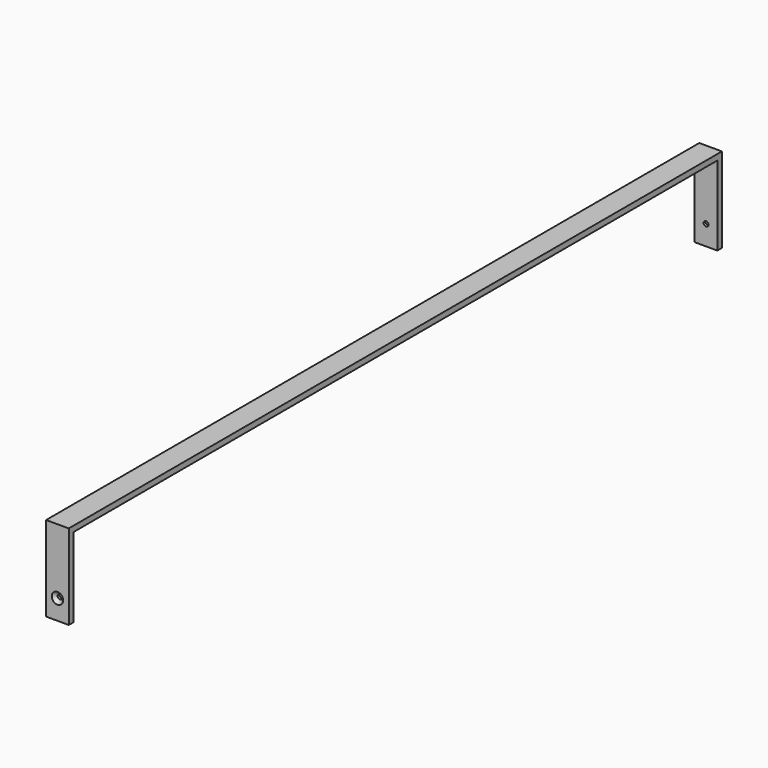
from build123d import *

# Parameters (mm, degrees)
F1_DEPTH       = 20
F3_D           = 8.5
F3_DEPTH       = 15
F3_CSINK_D     = 20
F3_CSINK_ANGLE = 90
F3_TIP         = 2.5536576309


# Not quite as in the source:
# - a pattern or mirror of a feature is missing from the dataset's text; its kind, count and spacing are read off the source's solid


with BuildPart() as f1:
    # F0 (on Right) → F1 (new body, symmetric)
    with BuildSketch(Plane.YZ):
        Polygon((720, 0), (0, 0), (-720, 0), (-720, -150), (-710, -150), (-710, -10), (0, -10), (710, -10), (710, -150), (720, -150), align=None)
    extrude(amount=F1_DEPTH, both=True)

    # F3
    with Locations(Plane.XZ.offset(720)):
        with Locations((0, -115)):
            f3 = CounterSinkHole(F3_D / 2, F3_CSINK_D / 2, depth=F3_DEPTH, counter_sink_angle=F3_CSINK_ANGLE)
            with Locations((0, 0, -(F3_DEPTH + F3_TIP / 2))):  # 118° drill point
                Cone(0, F3_D / 2, F3_TIP, mode=Mode.SUBTRACT)

    # F3_copies: F3 across plane
    add(f3.mirror(Plane.ZX), mode=Mode.SUBTRACT)


solid = f1.part
